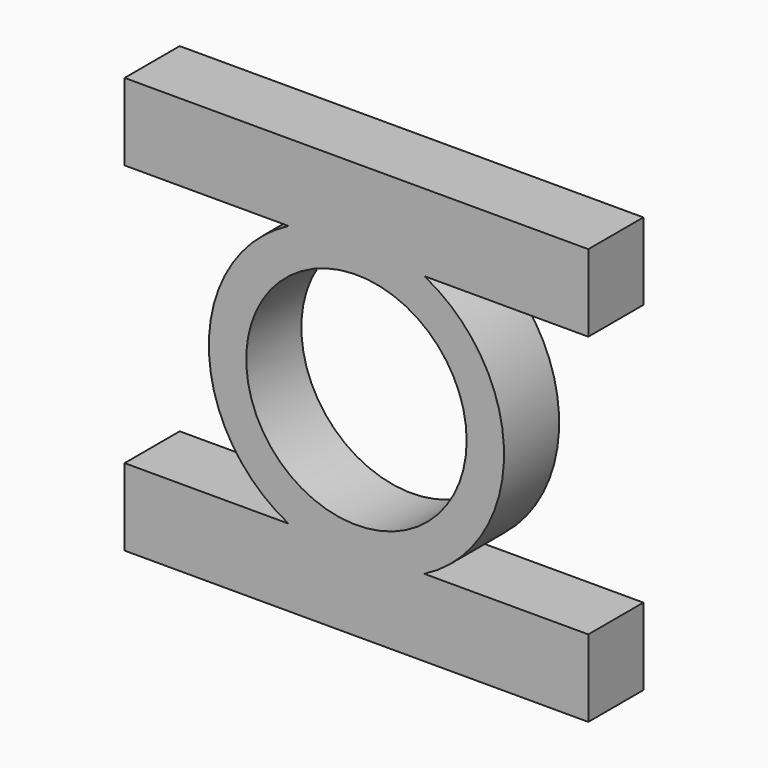
from build123d import *

# Parameters (mm, degrees)
F0_R     = 11.2
F1_DEPTH = 7


# Not quite as in the source:
# - a feature names something its author has since deleted; it is built from what else it names


with BuildPart() as f1:
    # F0 (on Front) → F1 (new body)
    with BuildSketch(Plane.XZ):
        with BuildLine():
            Line((-23.5628467053, 13.316613622), (-6.9041872543, 13.316613622))
            ThreePointArc((-6.9041872543, 13.316613622), (-15, 0), (-6.9041872543, -13.316613622))
            Line((-6.9041872543, -13.316613622), (-23.5628467053, -13.316613622))
            Line((-23.5628467053, -13.316613622), (-23.5628467053, -21.1474765092))
            Line((-23.5628467053, -21.1474765092), (0, -21.1474765092))
            Line((0, -21.1474765092), (23.5628467053, -21.1474765092))
            Line((23.5628467053, -21.1474765092), (23.5628467053, -13.316613622))
            Line((23.5628467053, -13.316613622), (6.9041872543, -13.316613622))
            ThreePointArc((6.9041872543, -13.316613622), (15, 0), (6.9041872543, 13.316613622))
            Line((6.9041872543, 13.316613622), (23.5628467053, 13.316613622))
            Line((23.5628467053, 13.316613622), (23.5628467053, 21.1474765092))
            Line((23.5628467053, 21.1474765092), (0, 21.1474765092))
            Line((0, 21.1474765092), (-23.5628467053, 21.1474765092))
            Line((-23.5628467053, 21.1474765092), (-23.5628467053, 13.316613622))
        make_face()
        Circle(F0_R, mode=Mode.SUBTRACT)
    extrude(amount=F1_DEPTH)


solid = f1.part
